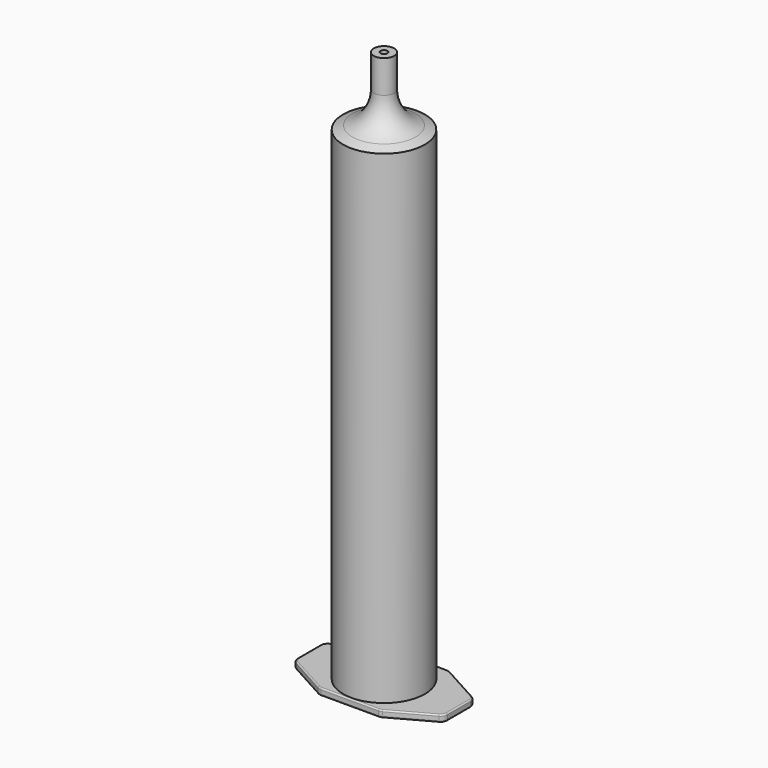
from build123d import *

# Parameters (mm, degrees)
F0_R          = 6
F0_R_2        = 5
F1_DEPTH      = 62
F1_DEPTH_BACK = 9
F6_DEPTH      = 1
F8_R          = 5
F9_DEPTH      = 1
F10_R         = 1
F11_R         = 0.2
F12_R         = 0.2


# Not quite as in the source:
# - a feature names something its author has since deleted; it is built from what else it names


with BuildPart() as f1:
    # F0 (on Top) → F1 (new body, two sides)
    with BuildSketch(Plane.XY) as f1_sk:
        Circle(F0_R)
        Circle(F0_R_2, mode=Mode.SUBTRACT)
    extrude(amount=F1_DEPTH)
    extrude(f1_sk.sketch, amount=-F1_DEPTH_BACK)

    # F2 (on Front) → F3 (revolve)
    with BuildSketch(Plane.XZ):
        with BuildLine():
            Line((6, 62), (4.6430466171, 62.5427813535))
            ThreePointArc((4.6430466171, 62.5427813535), (2.3596638473, 64.3820207615), (1.5, 67.1851648075))
            Line((1.5, 67.1851648075), (1.5, 72))
            Line((1.5, 72), (0.5, 72))
            Line((0.5, 72), (0.5, 63.8000000012))
            Line((0.5, 63.8000000012), (5, 62))
            Line((5, 62), (6, 62))
        make_face()
    revolve(axis=Axis((0, 0, 62.4439572394), (0, 0, 1)))

    # F5 (on offset) → F6 (join)
    with BuildSketch(Plane.XY.offset(-2)):
        with BuildLine():
            ThreePointArc((-3.5707142143, -3.5), (0, -5), (3.5707142143, -3.5))
            Line((3.5707142143, -3.5), (-3.5707142143, -3.5))
        make_face()
        with BuildLine():
            Line((-3.5707142143, 3.5), (3.5707142143, 3.5))
            ThreePointArc((3.5707142143, 3.5), (0, 5), (-3.5707142143, 3.5))
        make_face()
    extrude(amount=-F6_DEPTH)

    # F8 (on offset) → F9 (join)
    with BuildSketch(Plane(origin=(0, 0, -9), x_dir=(1, 0, 0), z_dir=(0, 0, -1))):
        Polygon((11, 2.7135847191), (4.4980677776, 6.3), (-4.4980677776, 6.3), (-11, 2.7135847191), (-11, -2.7135847191), (-4.4980677776, -6.3), (4.4980677776, -6.3), (11, -2.7135847191), align=None)
        Circle(F8_R, mode=Mode.SUBTRACT)
    extrude(amount=F9_DEPTH)

    # F10
    f10_edges = [f1.edges().sort_by_distance(p)[0] for p in [
        (11, -2.713585, -9.5),
        (4.498068, -6.3, -9.5),
        (11, 2.713585, -9.5),
        (-4.498068, -6.3, -9.5),
        (4.498068, 6.3, -9.5),
        (-11, -2.713585, -9.5),
        (-4.498068, 6.3, -9.5),
        (-11, 2.713585, -9.5),
    ]]
    fillet(f10_edges, radius=F10_R)

    # F11
    f11_edges = [f1.edges().sort_by_distance(p)[0] for p in [
        (-7.603269, -4.587195, -10),
        (-4.489932, -6.268408, -10),
        (0, -6.3, -10),
        (-11, 0, -10),
        (-10.861101, -2.631572, -10),
        (-10.861101, 2.631572, -10),
        (-7.603269, 4.587195, -10),
        (-4.489932, 6.268408, -10),
        (0, 6.3, -10),
        (4.489932, 6.268408, -10),
        (7.603269, 4.587195, -10),
        (7.603269, -4.587195, -10),
        (4.489932, -6.268408, -10),
        (10.861101, -2.631572, -10),
        (11, 0, -10),
        (10.861101, 2.631572, -10),
    ]]
    fillet(f11_edges, radius=F11_R)

    # F12
    f12_edges = [f1.edges().sort_by_distance(p)[0] for p in [
        (10.861101, -2.631572, -9),
        (11, 0, -9),
        (10.861101, 2.631572, -9),
        (7.603269, 4.587195, -9),
        (4.489932, 6.268408, -9),
        (0, 6.3, -9),
        (-4.489932, 6.268408, -9),
        (-10.861101, 2.631572, -9),
        (-7.603269, 4.587195, -9),
        (7.603269, -4.587195, -9),
        (0, -6.3, -9),
        (-11, 0, -9),
        (-10.861101, -2.631572, -9),
        (-4.489932, -6.268408, -9),
        (4.489932, -6.268408, -9),
        (-7.603269, -4.587195, -9),
    ]]
    fillet(f12_edges, radius=F12_R)


solid = f1.part
